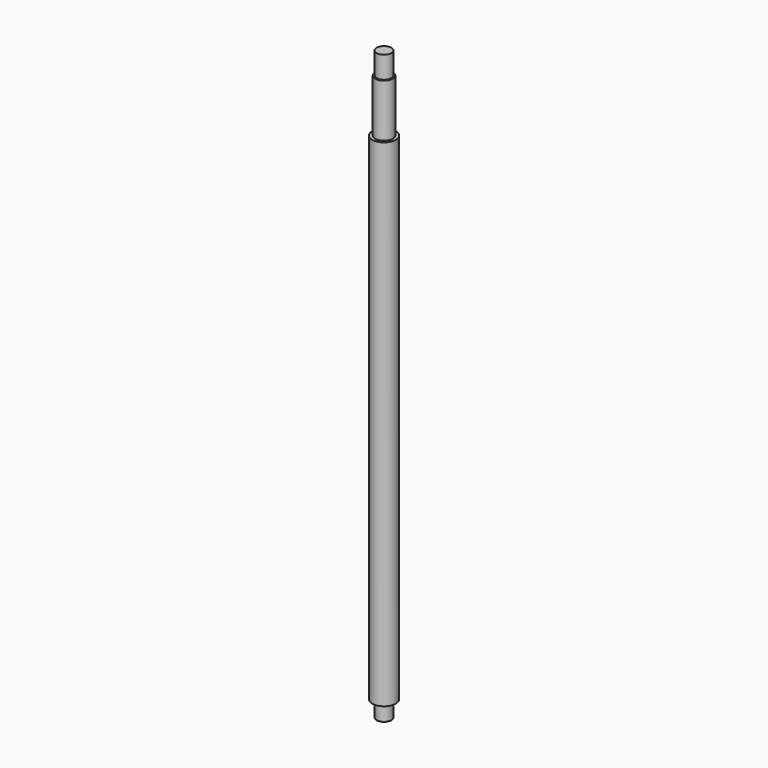
from build123d import *

# Parameters (mm, degrees)
F0_W   = 5
F0_H   = 15
F0_W_2 = 6
F0_H_2 = 22
F0_H_3 = 11
F3_R   = 0.2


# Not quite as in the source:
# - the program builds the solid bodies; features that only make, move or delete a surface that nothing else refers to are left out


with BuildPart() as f1:
    # F0 (on Front) → F1 (revolve)
    with BuildSketch(Plane.XZ):
        with Locations((2.5, 212.5)):
            Rectangle(F0_W, F0_H)
    revolve(axis=Axis((0, 0, -60.3163262457), (0, 0, -1)))



with BuildPart() as f1b:
    # F0 (on Front) → F1, piece 2 (revolve)
    with BuildSketch(Plane.XZ):
        with Locations((3, 180)):
            Rectangle(F0_W_2, F0_H_2)
        Polygon((0, 169), (0, 59.3673475087), (0, -169), (5, -169), (8.025, -169), (8.025, 169), (6, 169), align=None)
        with Locations((2.5, -174.5)):
            Rectangle(F0_W, F0_H_3)
    revolve(axis=Axis((0, 0, -60.3163262457), (0, 0, -1)))


with BuildPart() as f1_1:
    add(f1.part)

    add(f1b.part)  # F2 merges F1b
    # F0 (on Front) → F2 (revolve)
    with BuildSketch(Plane.XZ):
        Polygon((0, 205), (0, 191), (6, 191), (6, 205), (5, 205), align=None)
    revolve(axis=Axis((0, 0, 139.6836737543), (0, 0, 1)))

    # F3
    f3_edges = [f1_1.edges().sort_by_distance(p)[0] for p in [
        (-5, 0, -180),
    ]]
    fillet(f3_edges, radius=F3_R)


solid = f1_1.part
